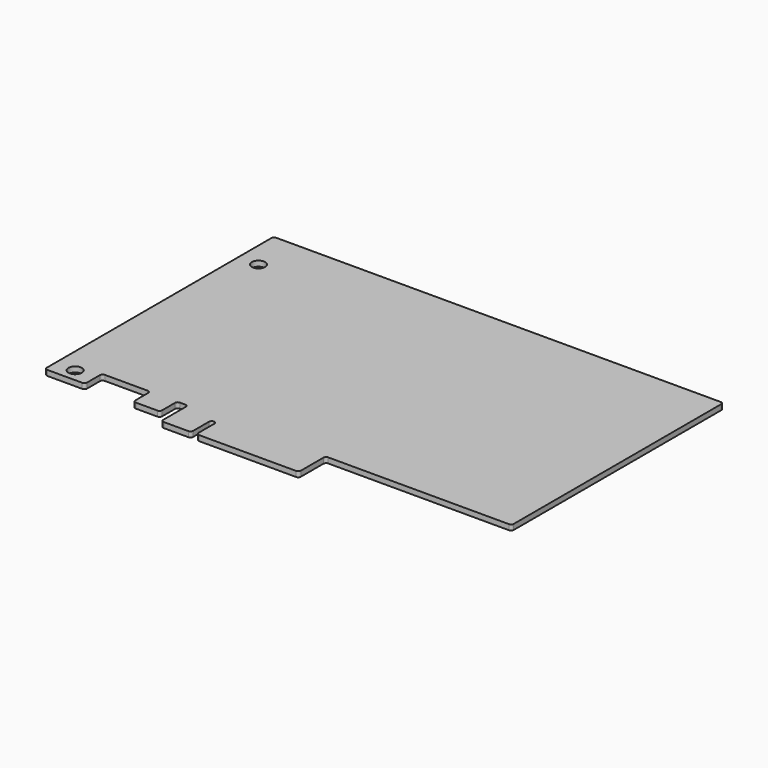
from build123d import *

# Parameters (mm, degrees)
F0_R     = 2.5
F1_DEPTH = 2
F2_R     = 0.99999


# Not quite as in the source:
# - a fillet or chamfer is up to 0.001 mm smaller than in the source, because OpenCascade refuses the exact size


with BuildPart() as f1:
    # F0 (on Top) → F1 (new body)
    with BuildSketch(Plane.XY):
        Polygon((-7.5, 101.8), (-7.5, -4.85), (7.5, -4.85), (7.5, 3.15), (25.5, 3.15), (25.5, -4.85), (35.5, -4.85), (35.5, 3.15), (39.5, 3.15), (39.5, -9.35), (50.65, -9.35), (50.65, 0), (52.65, 0), (52.65, -9.35), (90.8, -9.35), (90.8, 3.15), (160.15, 3.15), (160.15, 101.8), align=None)
        Circle(F0_R, mode=Mode.SUBTRACT)
        with Locations((0, 85.4)):
            Circle(F0_R, mode=Mode.SUBTRACT)
    extrude(amount=F1_DEPTH)

    # F2 (radius 1 in the source; OpenCascade refuses exactly that, so slightly less here)
    f2_edges = [f1.edges().sort_by_distance(p)[0] for p in [
        (-7.5, -4.85, 1),
        (7.5, -4.85, 1),
        (25.5, 3.15, 1),
        (25.5, -4.85, 1),
        (35.5, -4.85, 1),
        (39.5, 3.15, 1),
        (39.5, -9.35, 1),
        (50.65, -9.35, 1),
        (52.65, 0, 1),
        (52.65, -9.35, 1),
        (90.8, -9.35, 1),
        (-7.5, 101.8, 1),
        (160.15, 101.8, 1),
        (160.15, 3.15, 1),
        (90.8, 3.15, 1),
        (35.5, 3.15, 1),
        (7.5, 3.15, 1),
        (50.65, 0, 1),
    ]]
    fillet(f2_edges, radius=F2_R)


solid = f1.part
